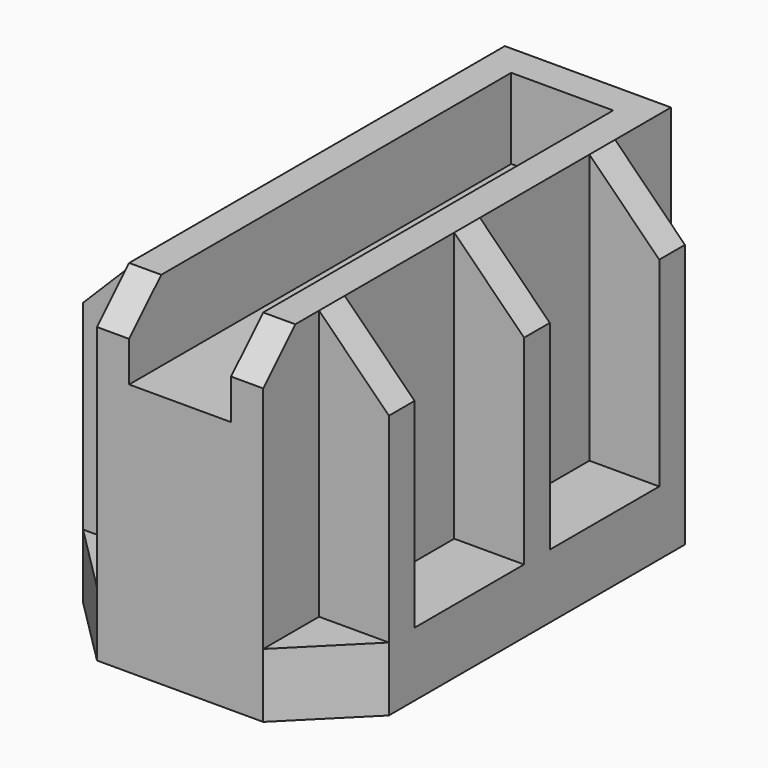
from build123d import *

# Parameters (mm, degrees)
F1_DEPTH  = 31.75
F2_T      = -4
F3_W      = 4
F3_H      = 10
F4_DEPTH  = 63.5
F6_DEPTH  = 8
F8_DEPTH  = 2
F11_DEPTH = 4
F13_DEPTH = 4
F14_W     = 12.7
F14_H     = 4
F15_DEPTH = 10
F16_SIZE  = 5
F17_R     = 2.15
F18_DEPTH = 25
F19_W     = 30.1
F19_H     = 4


# Not quite as in the source:
# - a pattern or mirror of a feature is missing from the dataset's text; its kind, count and spacing are read off the source's solid


with BuildPart() as f1:
    # F0 (on Front) → F1 (new body, symmetric)
    with BuildSketch(Plane.XZ):
        Polygon((-10.35, 0), (10.35, 0), (10.35, 31.575), (6.35, 31.575), (-6.35, 31.575), (-10.35, 31.575), align=None)
    extrude(amount=F1_DEPTH, both=True)

    # F2
    f2_openings = [f1.faces().sort_by_distance(p)[0] for p in [
        (0, 0, 0),
    ]]
    offset(amount=F2_T, openings=f2_openings)

    # F3 (on face) → F4 (join, through all)
    with BuildSketch(Plane.XZ.offset(31.75)):
        with Locations((-8.35, 36.575)):
            Rectangle(F3_W, F3_H)
        with Locations((8.35, 36.575)):
            Rectangle(F3_W, F3_H)
    extrude(amount=-F4_DEPTH)

    # F5 (on Top) → F6 (join)
    with BuildSketch(Plane.XY):
        Polygon((-19.05, -23.05), (-10.35, -31.75), (-10.35, 31.75), (-19.05, 23.05), align=None)
        Polygon((10.35, 31.75), (10.35, -31.75), (19.05, -23.05), (19.05, 23.05), align=None)
    extrude(amount=F6_DEPTH)

    # F7 (on Front) → F8 (join, symmetric)
    with BuildSketch(Plane.XZ):
        Polygon((-19.05, 8), (-10.35, 8), (-10.35, 41.575), (-19.05, 32.875), align=None)
        Polygon((10.35, 8), (19.05, 8), (19.05, 32.875), (10.35, 41.575), align=None)
    f8 = extrude(amount=F8_DEPTH, both=True)

    # F8_copies: F8 across plane
    add(f8.mirror(Plane(origin=(0, -10.525, 0), x_dir=(0, 0, -1), z_dir=(0, -1, 0))))

    # F10 (on plane+point) → F11 (join)
    with BuildSketch(Plane.XZ.offset(-23.05)):
        Polygon((10.35, 8), (19.05, 8), (19.05, 32.875), (10.35, 41.575), align=None)
        Polygon((-19.05, 32.875), (-19.05, 8), (-10.35, 8), (-10.35, 41.575), align=None)
    extrude(amount=F11_DEPTH)

    # F12 (on face) → F13 (cut)
    with BuildSketch(Plane(origin=(0, 0, 0), x_dir=(1, 0, 0), z_dir=(0, 0, -1))):
        Polygon((-8.6931457505, -27.75), (8.6931457505, -27.75), (15.05, -21.3931457505), (15.05, 21.3931457505), (8.6931457505, 27.75), (-8.6931457505, 27.75), (-15.05, 21.3931457505), (-15.05, -21.3931457505), align=None)
    extrude(amount=-F13_DEPTH, mode=Mode.SUBTRACT)

    # F14 (on face) → F15 (join, through all)
    with BuildSketch(Plane.XY.offset(31.575)):
        with Locations((0, 29.75)):
            Rectangle(F14_W, F14_H)
    extrude(amount=F15_DEPTH)

    # F16
    f16_edges = [f1.edges().sort_by_distance(p)[0] for p in [
        (8.35, -31.75, 41.575),
        (-8.35, -31.75, 41.575),
    ]]
    chamfer(f16_edges, length=F16_SIZE)

    # F17 (on face) → F18 (cut)
    with BuildSketch(Plane.XY.offset(31.575)):
        with Locations((0, -10.525)):
            Circle(F17_R)
    extrude(amount=-F18_DEPTH, mode=Mode.SUBTRACT)

    # F19 (on face) → F20 (join, up to the next surface of F1)
    with BuildSketch(Plane(origin=(0, 0, 0), x_dir=(1, 0, 0), z_dir=(0, 0, -1))):
        with Locations((0, -10.525)):
            Rectangle(F19_W, F19_H)
    extrude(until=Until.NEXT, dir=(0, 0, 1))


solid = f1.part
